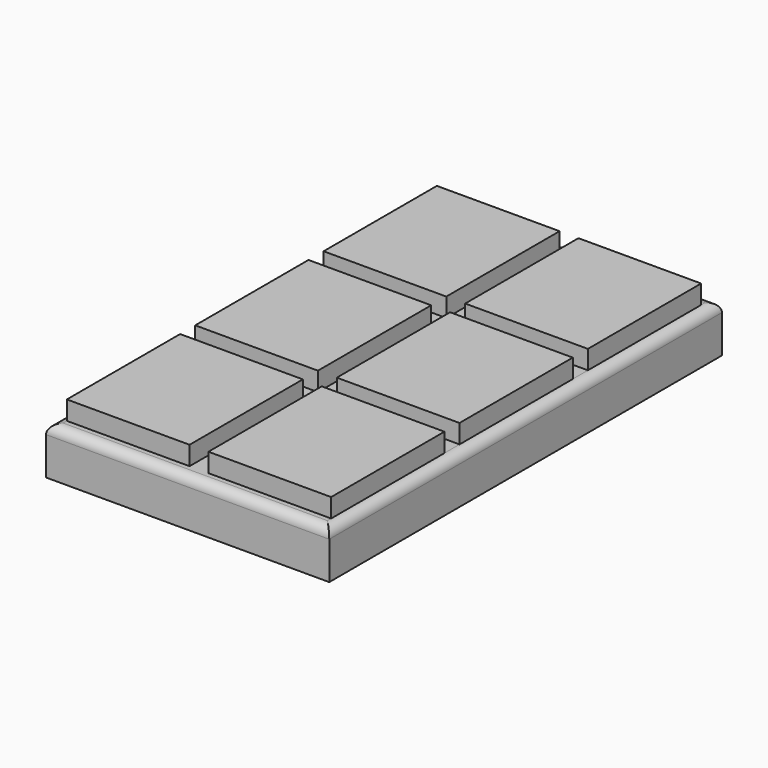
from build123d import *

# Parameters (mm, degrees)
F0_W     = 6.5
F0_H     = 15
F1_DEPTH = 7
F2_DEPTH = 5
F4_R     = 0.99999


# Not quite as in the source:
# - a fillet or chamfer is up to 0.001 mm smaller than in the source, because OpenCascade refuses the exact size
# - a feature names something its author has since deleted; it is built from what else it names


with BuildPart() as f1:
    # F0 (on Top) → F1 (new body)
    with BuildSketch(Plane.XY):
        with Locations((-4.25, 17)):
            Rectangle(F0_W, F0_H)
        with Locations((-10.75, 17)):
            Rectangle(F0_W, F0_H)
    extrude(amount=F1_DEPTH)


with BuildPart() as f1b:
    # F0 (on Top) → F1, piece 2 (new body)
    with BuildSketch(Plane.XY):
        with Locations((-10.75, 0)):
            Rectangle(F0_W, F0_H)
        with Locations((-4.25, 0)):
            Rectangle(F0_W, F0_H)
    extrude(amount=F1_DEPTH)


with BuildPart() as f1c:
    # F0 (on Top) → F1, piece 3 (new body)
    with BuildSketch(Plane.XY):
        with Locations((-4.25, -17)):
            Rectangle(F0_W, F0_H)
        with Locations((-10.75, -17)):
            Rectangle(F0_W, F0_H)
    extrude(amount=F1_DEPTH)


with BuildPart() as f1d:
    # F0 (on Top) → F1, piece 4 (new body)
    with BuildSketch(Plane.XY):
        with Locations((4.25, -17)):
            Rectangle(F0_W, F0_H)
        with Locations((10.75, -17)):
            Rectangle(F0_W, F0_H)
    extrude(amount=F1_DEPTH)


with BuildPart() as f1e:
    # F0 (on Top) → F1, piece 5 (new body)
    with BuildSketch(Plane.XY):
        with Locations((10.75, 0)):
            Rectangle(F0_W, F0_H)
        with Locations((4.25, 0)):
            Rectangle(F0_W, F0_H)
    extrude(amount=F1_DEPTH)


with BuildPart() as f1f:
    # F0 (on Top) → F1, piece 6 (new body)
    with BuildSketch(Plane.XY):
        with Locations((4.25, 17)):
            Rectangle(F0_W, F0_H)
        with Locations((10.75, 17)):
            Rectangle(F0_W, F0_H)
    extrude(amount=F1_DEPTH)


with BuildPart() as f2:
    # F0 (on Top) → F2 (new body)
    with BuildSketch(Plane.XY):
        Polygon((-7.5, 24.5), (-7.5, 26), (-15, 26), (-15, -26), (-7.5, -26), (-7.5, -24.5), (-14, -24.5), (-14, -9.5), (-7.5, -9.5), (-7.5, -7.5), (-14, -7.5), (-14, 7.5), (-7.5, 7.5), (-7.5, 9.5), (-14, 9.5), (-14, 24.5), align=None)
        Polygon((7.5, 24.5), (7.5, 26), (-7.5, 26), (-7.5, 24.5), (-1, 24.5), (-1, 9.5), (-7.5, 9.5), (-7.5, 7.5), (-1, 7.5), (-1, -7.5), (-7.5, -7.5), (-7.5, -9.5), (-1, -9.5), (-1, -24.5), (-7.5, -24.5), (-7.5, -26), (7.5, -26), (7.5, -24.5), (1, -24.5), (1, -9.5), (7.5, -9.5), (7.5, -7.5), (1, -7.5), (1, 7.5), (7.5, 7.5), (7.5, 9.5), (1, 9.5), (1, 24.5), align=None)
        Polygon((15, -26), (15, 26), (7.5, 26), (7.5, 24.5), (14, 24.5), (14, 9.5), (7.5, 9.5), (7.5, 7.5), (14, 7.5), (14, -7.5), (7.5, -7.5), (7.5, -9.5), (14, -9.5), (14, -24.5), (7.5, -24.5), (7.5, -26), align=None)
    extrude(amount=F2_DEPTH)


with BuildPart() as f1f_1:
    add(f1f.part)

    # F3: union F1b, F1c, F2, F1, F1d, F1e
    add(f1b.part)
    add(f1c.part)
    add(f2.part)
    add(f1.part)
    add(f1d.part)
    add(f1e.part)

    # F4 (radius 1 in the source; OpenCascade refuses exactly that, so slightly less here)
    f4_edges = [f1f_1.edges().sort_by_distance(p)[0] for p in [
        (-15, 0, 5),
        (0, -26, 5),
        (15, 0, 5),
        (0, 26, 5),
    ]]
    fillet(f4_edges, radius=F4_R)


solid = f1f_1.part
